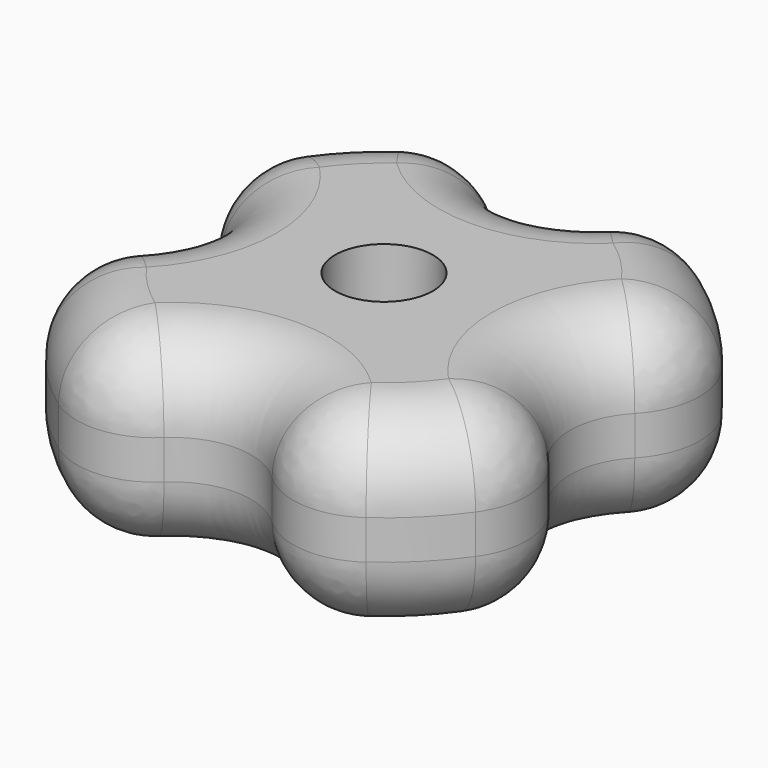
from build123d import *

# Parameters (mm, degrees)
F0_R     = 3.175
F1_DEPTH = 12.7
F2_R     = 5.08
F3_R     = 5.079


# Not quite as in the source:
# - a fillet or chamfer is up to 0.001 mm smaller than in the source, because OpenCascade refuses the exact size


with BuildPart() as f1:
    # F0 (on Top) → F1 (new body)
    with BuildSketch(Plane.XY):
        with BuildLine():
            ThreePointArc((-5.0239431117, -16.3924074074), (0, -12.065), (5.0239431117, -16.3924074074))
            ThreePointArc((5.0239431117, -16.3924074074), (12.1233457634, -12.1233457634), (16.3924074074, -5.0239431117))
            ThreePointArc((16.3924074074, -5.0239431117), (12.065, 0), (16.3924074074, 5.0239431117))
            ThreePointArc((16.3924074074, 5.0239431117), (12.1233457634, 12.1233457634), (5.0239431117, 16.3924074074))
            ThreePointArc((5.0239431117, 16.3924074074), (0, 12.065), (-5.0239431117, 16.3924074074))
            ThreePointArc((-5.0239431117, 16.3924074074), (-12.1233457634, 12.1233457634), (-16.3924074074, 5.0239431117))
            ThreePointArc((-16.3924074074, 5.0239431117), (-12.065, 0), (-16.3924074074, -5.0239431117))
            ThreePointArc((-16.3924074074, -5.0239431117), (-12.1233457634, -12.1233457634), (-5.0239431117, -16.3924074074))
        make_face()
        Circle(F0_R, mode=Mode.SUBTRACT)
    extrude(amount=F1_DEPTH)

    # F2
    f2_edges = [f1.edges().sort_by_distance(p)[0] for p in [
        (5.023943, 16.392407, 6.35),
        (-5.023943, 16.392407, 6.35),
        (16.392407, 5.023943, 6.35),
        (16.392407, -5.023943, 6.35),
        (5.023943, -16.392407, 6.35),
        (-5.023943, -16.392407, 6.35),
        (-16.392407, -5.023943, 6.35),
        (-16.392407, 5.023943, 6.35),
    ]]
    fillet(f2_edges, radius=F2_R)

    # F3 (radius 5.08 in the source; OpenCascade refuses exactly that, so slightly less here)
    f3_edges = [f1.edges().sort_by_distance(p)[0] for p in [
        (-6.666785, -14.874415, 12.7),
        (0, -12.065, 12.7),
        (6.666785, -14.874415, 12.7),
        (12.065, 0, 12.7),
        (14.874415, -6.666785, 12.7),
        (6.666785, 14.874415, 12.7),
        (0, 12.065, 12.7),
        (-14.874415, 6.666785, 12.7),
        (-6.666785, 14.874415, 12.7),
        (0, -12.065, 0),
        (-6.666785, -14.874415, 0),
        (6.666785, -14.874415, 0),
        (14.874415, -6.666785, 0),
        (12.065, 0, 0),
        (14.874415, 6.666785, 0),
        (-14.874415, -6.666785, 0),
        (-12.065, 0, 0),
        (-14.874415, 6.666785, 0),
        (-6.666785, 14.874415, 0),
        (0, 12.065, 0),
    ]]
    fillet(f3_edges, radius=F3_R)


solid = f1.part
